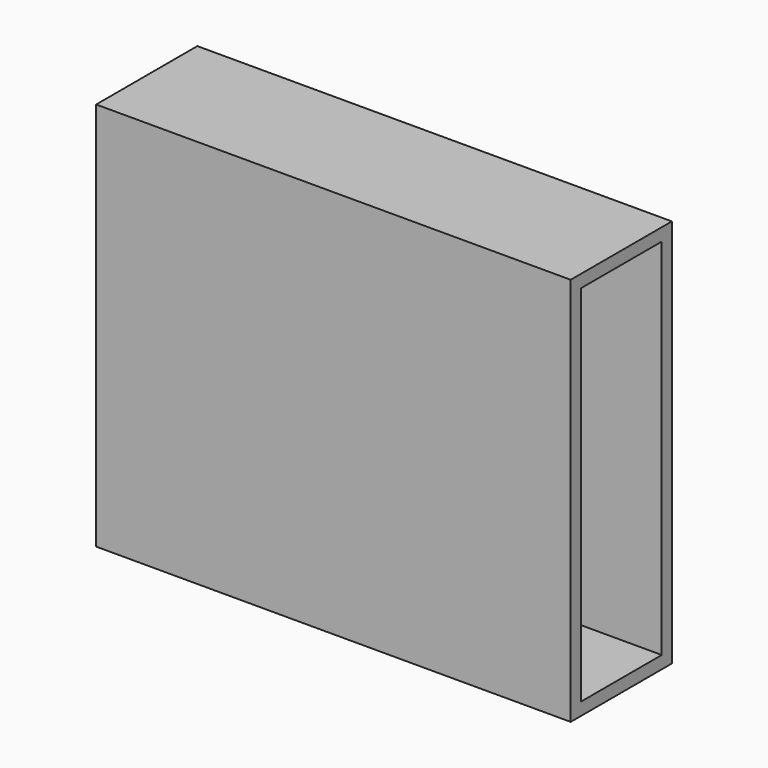
from build123d import *

# Parameters (mm, degrees)
F0_W         = 95.3032001853
F0_H         = 78.1703665853
F1_DEPTH     = 25.4
F2_T         = -2.54
F3_W         = 5.7767406106
F3_H         = 42.3835292459
F4_DEPTH     = 3.175
F5_W         = 5.7767406106
F5_H         = 42.3835292459
F6_DEPTH     = 3.175
F7_T1_DEPTH  = 66.0677355788
F7_T3_DEPTH  = 66.8133734297
F7_T8_DEPTH  = 84.3633291385
F7_T13_DEPTH = 84.3633291385
F8_T1_DEPTH  = 33.1027333037
F8_T6_ANGLE  = 211.2479562886
F8_T12_ANGLE = 207.4140629141
F8_T15_DEPTH = 67.9213053823


# Not quite as in the source:
# - a fillet or chamfer that OpenCascade refuses, or shapes differently, is made with other operations: its cross-section is extruded or revolved along the edge and cut away or added


with BuildPart() as f1:
    # F0 (on Front) → F1 (new body)
    with BuildSketch(Plane.XZ):
        with Locations((47.6516000926, 39.0851832926)):
            Rectangle(F0_W, F0_H)
    extrude(amount=F1_DEPTH)

    # F2
    f2_openings = [f1.faces().sort_by_distance(p)[0] for p in [
        (95.3032, -12.7, 39.085183),
    ]]
    offset(amount=F2_T, openings=f2_openings)

    # F3 (on face) → F4 (join)
    with BuildSketch(Plane(origin=(0, 0, 0), x_dir=(-1, 0, 0), z_dir=(0, 1, 0))):
        with Locations((-77.4001292884, 39.3448248506)):
            Rectangle(F3_W, F3_H)
    extrude(amount=F4_DEPTH)

    # F5 (on face) → F6 (join)
    with BuildSketch(Plane(origin=(0, 3.175, 0), x_dir=(-1, 0, 0), z_dir=(0, 1, 0))):
        Polygon((-74.5117589831, 60.5365894735), (-74.5117589831, 18.1530602276), (-19.4716006517, 18.1530602276), (-19.4716006517, 60.6743656099), (-80.2884995937, 60.6743656099), (-80.2884995937, 60.5365894735), align=None)
        with Locations((-77.4001292884, 39.3448248506)):
            Rectangle(F5_W, F5_H)
    extrude(amount=F6_DEPTH)

    # F7: fillet of radius 5.08 on 3 edges, made by hand

    # F7_s2 → F7_t1 (cut)
    with BuildSketch(Plane.XY.offset(6.3798451294)):
        with BuildLine():
            ThreePointArc((19.4716006517, 6.35), (21.3410803596, 4.0428865162), (24.180886691, 3.175))
            Line((24.180886691, 3.175), (19.4716006517, 3.175))
            Line((19.4716006517, 3.175), (19.4716006517, 6.35))
        make_face()
    extrude(amount=F7_T1_DEPTH, mode=Mode.SUBTRACT)

    # F7_s4 → F7_t3 (cut)
    with BuildSketch(Plane.YZ.offset(7.6983855535)):
        with BuildLine():
            ThreePointArc((3.175, 22.8623462669), (4.0428865162, 20.0225399355), (6.35, 18.1530602276))
            Line((6.35, 18.1530602276), (3.175, 18.1530602276))
            Line((3.175, 18.1530602276), (3.175, 22.8623462669))
        make_face()
    extrude(amount=F7_T3_DEPTH, mode=Mode.SUBTRACT)


with BuildPart() as f7_tool6:
    # F7_s7 → F7_t8 (new body)
    with BuildSketch(Plane.YZ.offset(7.6983855535)):
        with BuildLine():
            ThreePointArc((6.35, 60.6743656099), (4.0428865162, 58.804885902), (3.175, 55.9650795706))
            Line((3.175, 55.9650795706), (3.175, 60.6743656099))
            Line((3.175, 60.6743656099), (6.35, 60.6743656099))
        make_face()
    extrude(amount=F7_T8_DEPTH)

    split(bisect_by=Plane.XY.offset(60.5365894735), keep=Keep.TOP)


with BuildPart() as f1_1:
    add(f1.part)

    # F7_t5: cut F7_tool6
    add(f7_tool6.part, mode=Mode.SUBTRACT)


with BuildPart() as f7_tool11:
    # F7_s12 → F7_t13 (new body)
    with BuildSketch(Plane.YZ.offset(7.6983855535)):
        with BuildLine():
            ThreePointArc((6.35, 60.6743656099), (4.0428865162, 58.804885902), (3.175, 55.9650795706))
            Line((3.175, 55.9650795706), (3.175, 60.6743656099))
            Line((3.175, 60.6743656099), (6.35, 60.6743656099))
        make_face()
    extrude(amount=F7_T13_DEPTH)

    split(bisect_by=Plane.YZ.offset(74.5117589831), keep=Keep.BOTTOM)


with BuildPart() as f1_2:
    add(f1_1.part)

    # F7_t10: cut F7_tool11
    add(f7_tool11.part, mode=Mode.SUBTRACT)

    # F8: fillet of radius 5.08 on 2 edges, made by hand

    # F8_s2 → F8_t1 (join)
    with BuildSketch(Plane.XY.offset(22.8623462669)):
        with BuildLine():
            ThreePointArc((69.4317589831, 3.175), (73.0238614316, 1.6871024484), (74.5117589831, -1.905))
            Line((74.5117589831, -1.905), (74.5117589831, 3.175))
            Line((74.5117589831, 3.175), (69.4317589831, 3.175))
        make_face()
    extrude(amount=F8_T1_DEPTH)


with BuildPart() as f8_tool4:
    # F8_s5 → F8_t6 (revolve)
    with BuildSketch(Plane.XY.offset(22.8623462668)):
        with BuildLine():
            ThreePointArc((69.4317589831, 3.175), (73.0238614316, 1.6871024484), (74.5117589831, -1.905))
            Line((74.5117589831, -1.905), (74.5117589831, 3.175))
            Line((74.5117589831, 3.175), (69.4317589831, 3.175))
        make_face()
    revolve(axis=Axis((74.5117589831, 8.2549999999, 22.8623462668), (1, 0, 0)), revolution_arc=F8_T6_ANGLE)

    split(bisect_by=Plane.XZ.offset(-6.35), keep=Keep.TOP)

    split(bisect_by=Plane.XY.offset(18.1530602276), keep=Keep.TOP)


with BuildPart() as f1_3:
    add(f1_2.part)

    # F8_t3: union F8_tool4
    add(f8_tool4.part)


with BuildPart() as f8_tool10:
    # F8_s11 → F8_t12 (revolve)
    with BuildSketch(Plane.XY.offset(55.9650795707)):
        with BuildLine():
            ThreePointArc((69.4317589831, 3.175), (73.0238614316, 1.6871024484), (74.5117589831, -1.905))
            Line((74.5117589831, -1.905), (74.5117589831, 3.175))
            Line((74.5117589831, 3.175), (69.4317589831, 3.175))
        make_face()
    revolve(axis=Axis((74.5117589831, 8.2549999999, 55.9650795707), (-1, 0, 0)), revolution_arc=F8_T12_ANGLE)

    split(bisect_by=Plane.XZ.offset(-6.35), keep=Keep.TOP)

    split(bisect_by=Plane.XY.offset(60.5365894735), keep=Keep.BOTTOM)


with BuildPart() as f1_4:
    add(f1_3.part)

    # F8_t9: union F8_tool10
    add(f8_tool10.part)

    # F8_s16 → F8_t15 (cut)
    with BuildSketch(Plane.XY.offset(5.4530602276)):
        with BuildLine():
            ThreePointArc((75.2084995937, 6.35), (78.8006020422, 4.8621024484), (80.2884995937, 1.27))
            Line((80.2884995937, 1.27), (80.2884995937, 6.35))
            Line((80.2884995937, 6.35), (75.2084995937, 6.35))
        make_face()
    extrude(amount=F8_T15_DEPTH, mode=Mode.SUBTRACT)


solid = f1_4.part
